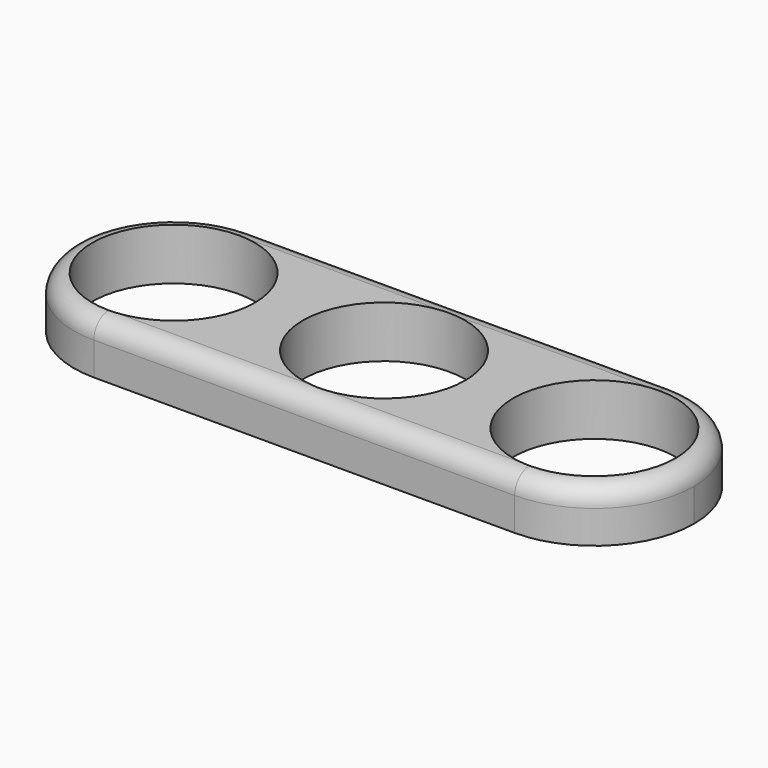
from build123d import *

# Parameters (mm, degrees)
F0_R        = 10.9982
F0_R_2      = 11
F1_DEPTH    = 7
F2_T1_DEPTH = 57
F2_T4_ANGLE = 180
F2_T6_ANGLE = 180


# Not quite as in the source:
# - a fillet or chamfer that OpenCascade refuses, or shapes differently, is made with other operations: its cross-section is extruded or revolved along the edge and cut away or added


with BuildPart() as f1:
    # F0 (on Top) → F1 (new body)
    with BuildSketch(Plane.XY):
        with BuildLine():
            ThreePointArc((-28.5, 13.5), (-18.954058454, 9.545941546), (-15, 0))
            ThreePointArc((-15, 0), (-18.954058454, -9.545941546), (-28.5, -13.5))
            Line((-28.5, -13.5), (28.5, -13.5))
            ThreePointArc((28.5, -13.5), (15, 0), (28.5, 13.5))
            Line((28.5, 13.5), (-28.5, 13.5))
        make_face()
        Circle(F0_R, mode=Mode.SUBTRACT)
        with BuildLine():
            ThreePointArc((-28.5, -13.5), (-18.954058454, -9.545941546), (-15, 0))
            ThreePointArc((-15, 0), (-18.954058454, 9.545941546), (-28.5, 13.5))
            ThreePointArc((-28.5, 13.5), (-42, 0), (-28.5, -13.5))
        make_face()
        with Locations((-28.5, 0)):
            Circle(F0_R_2, mode=Mode.SUBTRACT)
        with BuildLine():
            ThreePointArc((42, 0), (38.045941546, 9.545941546), (28.5, 13.5))
            ThreePointArc((28.5, 13.5), (15, 0), (28.5, -13.5))
            ThreePointArc((28.5, -13.5), (38.045941546, -9.545941546), (42, 0))
        make_face()
        with Locations((28.5, 0)):
            Circle(F0_R_2, mode=Mode.SUBTRACT)
    extrude(amount=F1_DEPTH)

    # F2: fillet of radius 2.54 on 4 edges, made by hand

    # F2_s2 → F2_t1 (cut)
    with BuildSketch(Plane.YZ.offset(-28.5)):
        with BuildLine():
            ThreePointArc((13.5, 4.46), (12.7560512242, 6.2560512242), (10.96, 7))
            Line((10.96, 7), (13.5, 7))
            Line((13.5, 7), (13.5, 4.46))
        make_face()
        with BuildLine():
            ThreePointArc((-13.5, 4.46), (-12.7560512242, 6.2560512242), (-10.96, 7))
            Line((-10.96, 7), (-13.5, 7))
            Line((-13.5, 7), (-13.5, 4.46))
        make_face()
    extrude(amount=F2_T1_DEPTH, mode=Mode.SUBTRACT)

    # F2_s3 → F2_t4 (revolve, cut)
    with BuildSketch(Plane.YZ.offset(-28.5)):
        with BuildLine():
            ThreePointArc((13.5, 4.46), (12.7560512242, 6.2560512242), (10.96, 7))
            Line((10.96, 7), (13.5, 7))
            Line((13.5, 7), (13.5, 4.46))
        make_face()
    revolve(axis=Axis((-28.5, 0, 7), (0, 0, 1)), revolution_arc=F2_T4_ANGLE, mode=Mode.SUBTRACT)

    # F2_s5 → F2_t6 (revolve, cut)
    with BuildSketch(Plane.YZ.offset(28.5)):
        with BuildLine():
            ThreePointArc((-13.5, 4.46), (-12.7560512242, 6.2560512242), (-10.96, 7))
            Line((-10.96, 7), (-13.5, 7))
            Line((-13.5, 7), (-13.5, 4.46))
        make_face()
    revolve(axis=Axis((28.5, 0, 7), (0, 0, 1)), revolution_arc=F2_T6_ANGLE, mode=Mode.SUBTRACT)


solid = f1.part
